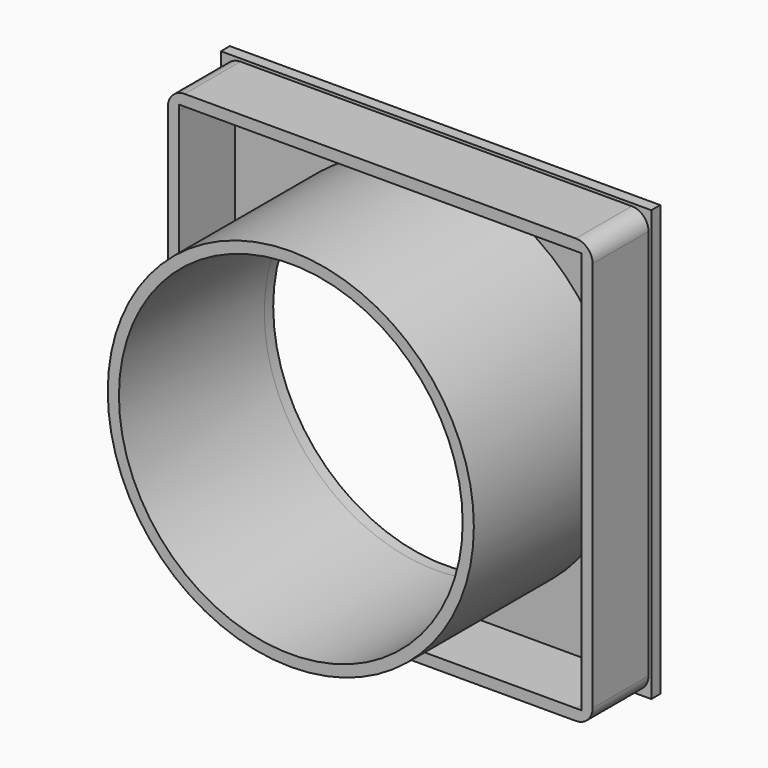
from build123d import *

# Parameters (mm, degrees)
F0_W     = 154
F0_H     = 154
F1_DEPTH = 4
F3_DEPTH = 25
F4_R     = 65.5
F4_R_2   = 61.5
F5_DEPTH = 65
F6_DEPTH = 88.2


# Not quite as in the source:
# - ends of sketch curves that miss each other by under 0.0002 mm in the source are joined


with BuildPart() as f1:
    # F0 (on Front) → F1 (new body)
    with BuildSketch(Plane.XZ):
        Rectangle(F0_W, F0_H)
    extrude(amount=-F1_DEPTH)

    # F2 (on face) → F3 (join)
    with BuildSketch(Plane.XZ):
        with BuildLine():
            ThreePointArc((-76, -70), (-74.2426406871, -74.2426406871), (-70, -76))
            Line((-70, -76), (70, -76))
            ThreePointArc((70, -76), (74.2426406871, -74.2426406871), (76, -70))
            Line((76, -70), (76, 70))
            ThreePointArc((76, 70), (74.2426406871, 74.2426406871), (70, 76))
            Line((70, 76), (-70, 76))
            ThreePointArc((-70, 76), (-74.2426406871, 74.2426406871), (-76, 70))
            Line((-76, 70), (-76, -70))
        make_face()
        Polygon((-71.9999969006, 71.9999969006), (-70, 71.9999969006), (70, 72), (71.9999969006, 71.9999969006), (71.9999969006, 70), (72, -70), (71.9999969006, -71.9999969006), (70, -71.9999969006), (-70, -72), (-71.9999969006, -71.9999969006), (-71.9999969006, -70), (-72, 70), align=None, mode=Mode.SUBTRACT)
    extrude(amount=F3_DEPTH)

    # F4 (on face) → F5 (join)
    with BuildSketch(Plane.XZ):
        Circle(F4_R)
        Circle(F4_R_2, mode=Mode.SUBTRACT)
    extrude(amount=F5_DEPTH)

    # F6 (cut): a face of the model
    f6_faces = [f1.faces().sort_by_distance(p)[0] for p in [
        (0, 0, 0),
    ]]
    extrude(f6_faces, amount=-F6_DEPTH, mode=Mode.SUBTRACT)


solid = f1.part
